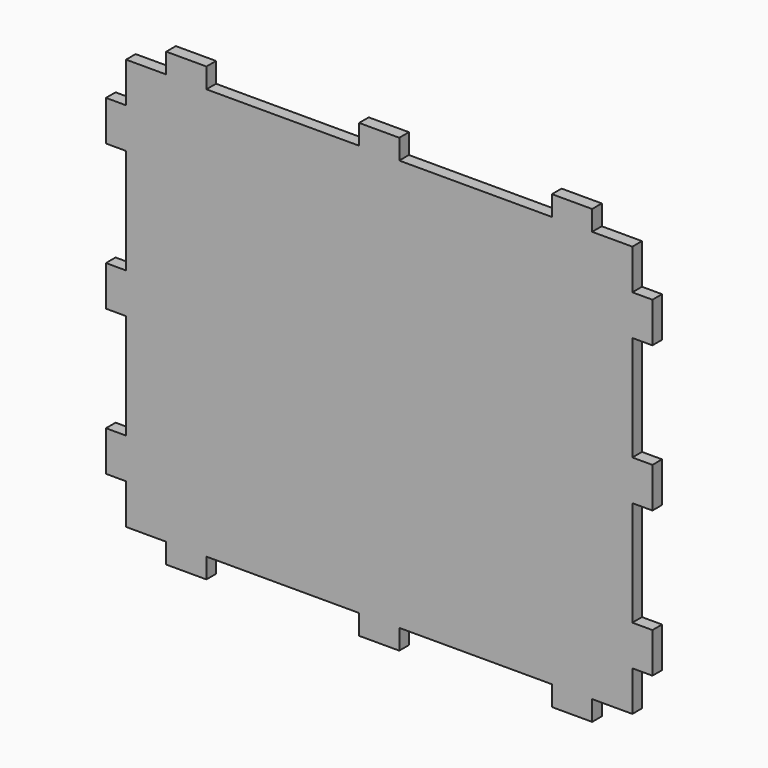
from build123d import *

# Parameters (mm, degrees)
F0_W     = 6.35
F0_H     = 12.7
F0_W_2   = 12.7
F0_H_2   = 6.35
F1_DEPTH = 3.81


# Not quite as in the source:
# - a feature names something its author has since deleted; it is built from what else it names


with BuildPart() as f1:
    # F0 (on Front) → F1 (new body)
    with BuildSketch(Plane.XZ):
        with Locations((-354.6769669852, 49.3793434303)):
            Rectangle(F0_W, F0_H)
        with Locations((-361.0269669852, 49.3793434303)):
            Rectangle(F0_W, F0_H)
        Polygon((-332.4519669852, -61.5706565697), (-284.2019669852, -61.5706565697), (-284.2019669852, -55.2206565697), (-277.8519669852, -55.2206565697), (-277.8519669852, 62.0793434303), (-284.2019669852, 62.0793434303), (-284.2019669852, 68.4293434303), (-332.4519669852, 68.4293434303), (-332.4519669852, 62.0793434303), (-345.1519669852, 62.0793434303), (-345.1519669852, 68.4293434303), (-357.8519669852, 68.4293434303), (-357.8519669852, 55.7293434303), (-351.5019669852, 55.7293434303), (-351.5019669852, 43.0293434303), (-357.8519669852, 43.0293434303), (-357.8519669852, 9.7793434303), (-351.5019669852, 9.7793434303), (-351.5019669852, -2.9206565697), (-357.8519669852, -2.9206565697), (-357.8519669852, -36.1706565697), (-351.5019669852, -36.1706565697), (-351.5019669852, -48.8706565697), (-357.8519669852, -48.8706565697), (-357.8519669852, -61.5706565697), (-345.1519669852, -61.5706565697), (-345.1519669852, -55.2206565697), (-332.4519669852, -55.2206565697), align=None)
        with Locations((-338.8019669852, 65.2543434303)):
            Rectangle(F0_W_2, F0_H_2)
        with Locations((-338.8019669852, 71.6043434303)):
            Rectangle(F0_W_2, F0_H_2)
        Polygon((-210.5519669852, -61.5706565697), (-197.8519669852, -61.5706565697), (-197.8519669852, -48.8706565697), (-204.2019669852, -48.8706565697), (-204.2019669852, -36.1706565697), (-197.8519669852, -36.1706565697), (-197.8519669852, -2.9206565697), (-204.2019669852, -2.9206565697), (-204.2019669852, 9.7793434303), (-197.8519669852, 9.7793434303), (-197.8519669852, 43.0293434303), (-204.2019669852, 43.0293434303), (-204.2019669852, 55.7293434303), (-197.8519669852, 55.7293434303), (-197.8519669852, 68.4293434303), (-210.5519669852, 68.4293434303), (-210.5519669852, 62.0793434303), (-223.2519669852, 62.0793434303), (-223.2519669852, 68.4293434303), (-271.5019669852, 68.4293434303), (-271.5019669852, 62.0793434303), (-277.8519669852, 62.0793434303), (-277.8519669852, -55.2206565697), (-271.5019669852, -55.2206565697), (-271.5019669852, -61.5706565697), (-223.2519669852, -61.5706565697), (-223.2519669852, -55.2206565697), (-210.5519669852, -55.2206565697), align=None)
        Polygon((-284.2019669852, 68.4293434303), (-277.8519669852, 68.4293434303), (-271.5019669852, 68.4293434303), (-271.5019669852, 74.7793434303), (-284.2019669852, 74.7793434303), align=None)
        with Locations((-274.6769669852, 65.2543434303)):
            Rectangle(F0_W, F0_H_2)
        with Locations((-281.0269669852, 65.2543434303)):
            Rectangle(F0_W, F0_H_2)
        with Locations((-216.9019669852, 71.6043434303)):
            Rectangle(F0_W_2, F0_H_2)
        with Locations((-216.9019669852, 65.2543434303)):
            Rectangle(F0_W_2, F0_H_2)
        with Locations((-354.6769669852, 3.4293434303)):
            Rectangle(F0_W, F0_H)
        with Locations((-361.0269669852, 3.4293434303)):
            Rectangle(F0_W, F0_H)
        with Locations((-361.0269669852, -42.5206565697)):
            Rectangle(F0_W, F0_H)
        with Locations((-338.8019669852, -64.7456565697)):
            Rectangle(F0_W_2, F0_H_2)
        with Locations((-354.6769669852, -42.5206565697)):
            Rectangle(F0_W, F0_H)
        with Locations((-338.8019669852, -58.3956565697)):
            Rectangle(F0_W_2, F0_H_2)
        with Locations((-281.0269669852, -58.3956565697)):
            Rectangle(F0_W, F0_H_2)
        with Locations((-274.6769669852, -58.3956565697)):
            Rectangle(F0_W, F0_H_2)
        Polygon((-271.5019669852, -67.9206565697), (-271.5019669852, -61.5706565697), (-277.8519669852, -61.5706565697), (-284.2019669852, -61.5706565697), (-284.2019669852, -67.9206565697), align=None)
        with Locations((-216.9019669852, -64.7456565697)):
            Rectangle(F0_W_2, F0_H_2)
        with Locations((-216.9019669852, -58.3956565697)):
            Rectangle(F0_W_2, F0_H_2)
        with Locations((-201.0269669852, -42.5206565697)):
            Rectangle(F0_W, F0_H)
        with Locations((-194.6769669852, -42.5206565697)):
            Rectangle(F0_W, F0_H)
        with Locations((-201.0269669852, 3.4293434303)):
            Rectangle(F0_W, F0_H)
        with Locations((-194.6769669852, 3.4293434303)):
            Rectangle(F0_W, F0_H)
        with Locations((-201.0269669852, 49.3793434303)):
            Rectangle(F0_W, F0_H)
        with Locations((-194.6769669852, 49.3793434303)):
            Rectangle(F0_W, F0_H)
    extrude(amount=F1_DEPTH)


solid = f1.part
